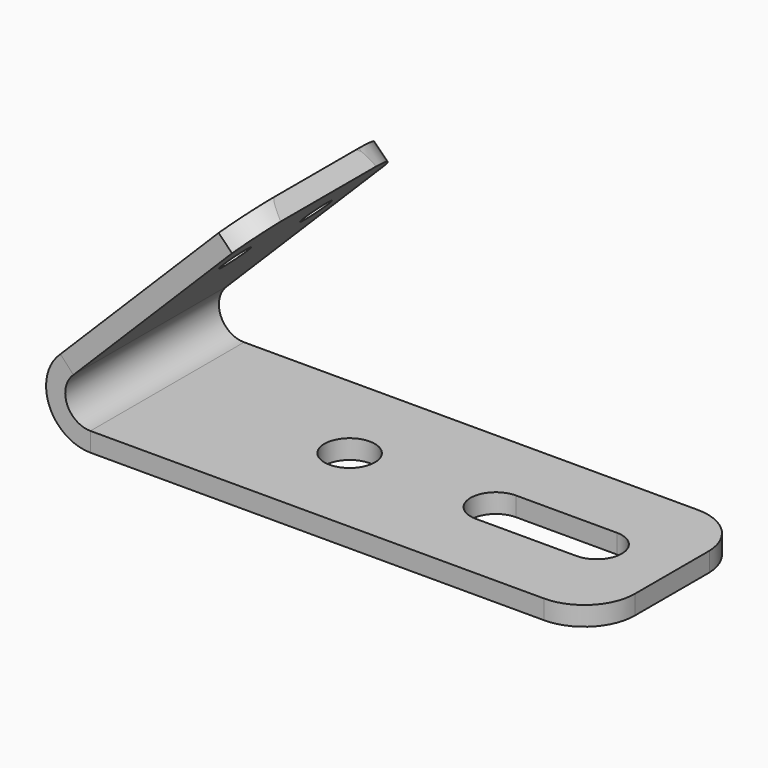
from build123d import *

# Parameters (mm, degrees)
F0_R     = 63.5
F1_DEPTH = 48.26
F3_DEPTH = 483.87
F6_DEPTH = 483.87
F7_R     = 38.1
F8_DEPTH = 48.26


# Not quite as in the source:
# - a feature of the source that left no trace in its solid (it failed there, or was rolled back) is left out


with BuildPart() as f1:
    # F0 (on Top) → F1 (new body)
    with BuildSketch(Plane.XY):
        with BuildLine():
            Line((685.9299561556, 239.0631011906), (-457.2, 239.0631011906))
            Line((-457.2, 239.0631011906), (-457.2, -244.8068988094))
            Line((-457.2, -244.8068988094), (685.9299561556, -244.8068988094))
            ThreePointArc((685.9299561556, -244.8068988094), (775.6484959021, -207.5635683113), (812.8, -117.8069653))
            Line((812.8, -117.8069653), (812.8, 117.8069653))
            ThreePointArc((812.8, 117.8069653), (773.6782588688, 203.8739685808), (685.9299561556, 239.0631011906))
        make_face()
        Circle(F0_R, mode=Mode.SUBTRACT)
        with BuildLine():
            ThreePointArc((368.4297373828, -63.5), (304.9297373818, -0.0001093866), (368.4295186092, 63.5))
            Line((368.4295186092, 63.5), (622.4297373818, 63.5))
            ThreePointArc((622.4297373818, 63.5), (685.9299561555, 0.000109387), (622.4299561555, -63.5))
            Line((622.4299561555, -63.5), (368.4297373828, -63.5))
        make_face(mode=Mode.SUBTRACT)
    extrude(amount=F1_DEPTH)


with BuildPart() as f3:
    # F2 (on face) → F3 (new body)
    with BuildSketch(Plane.XZ.offset(244.8068988094)):
        with BuildLine():
            Line((-500.1199795269, 158.55877517), (-532.7391639674, 194.1258442992))
            ThreePointArc((-532.7391639674, 194.1258442992), (-561.3525428371, 71.2316713821), (-457.2, 0))
            Line((-457.2, 0), (-457.2, 48.26))
            ThreePointArc((-457.2, 48.26), (-516.3775811575, 88.732540558), (-500.1199795269, 158.55877517))
        make_face()
    extrude(amount=-F3_DEPTH)


with BuildPart() as f6:
    # F5 (on face) → F6 (new body)
    with BuildSketch(Plane.XZ.offset(244.8068988094)):
        Polygon((-83.7263579139, 643.1386503526), (-532.7391639674, 194.1258442992), (-500.1199795269, 158.55877517), (-51.1071734735, 607.5715812234), align=None)
    extrude(amount=-F6_DEPTH)

    # F7 (on face) → F8 (cut)
    with BuildSketch(Plane(origin=(-363.4325041333, 0, 363.4325041333), x_dir=(0, -1, 0), z_dir=(-0.7071067812, 0, 0.7071067812))):
        with BuildLine():
            Line((244.8068988094, 395.5642254625), (130.5068988094, 395.5642254625))
            ThreePointArc((130.5068988094, 395.5642254625), (197.9551452431, 376.1733981804), (244.8068988094, 323.9222420455))
            Line((244.8068988094, 323.9222420455), (244.8068988094, 395.5642254625))
        make_face()
        with Locations((-124.7631011906, 205.0642254625)):
            Circle(F7_R)
        with Locations((130.5068988094, 205.0642254625)):
            Circle(F7_R)
        with BuildLine():
            Line((-134.0684582131, 395.2228624783), (-124.7631011906, 395.5642254625))
            ThreePointArc((-124.7631011906, 395.5642254625), (-129.4189093375, 395.4788560238), (-134.0684582131, 395.2228624783))
        make_face()
        with BuildLine():
            ThreePointArc((-134.0684582131, 395.2228624783), (-129.4189093375, 395.4788560238), (-124.7631011906, 395.5642254625))
            Line((-124.7631011906, 395.5642254625), (-239.0631011906, 395.5642254625))
            Line((-239.0631011906, 395.5642254625), (-239.0631011906, 323.9222420455))
            ThreePointArc((-239.0631011906, 323.9222420455), (-196.110951121, 373.6284168424), (-134.0684582131, 395.2228624783))
        make_face()
    extrude(amount=-F8_DEPTH, mode=Mode.SUBTRACT)


solid = Compound([f1.part, f3.part, f6.part])
